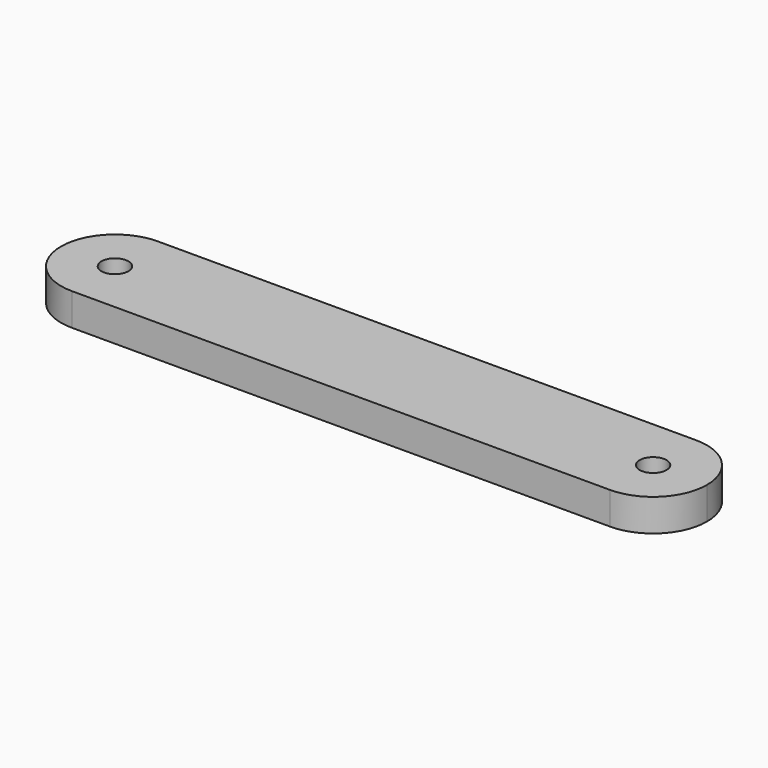
from build123d import *

# Parameters (mm, degrees)
F0_W     = 30.48
F0_H     = 5.08
F0_R     = 0.635
F1_DEPTH = 1.524
F2_R     = 2.53999


# Not quite as in the source:
# - a fillet or chamfer is up to 0.001 mm smaller than in the source, because OpenCascade refuses the exact size


with BuildPart() as f1:
    # F0 (on Top) → F1 (new body)
    with BuildSketch(Plane.XY):
        with Locations((15.24, 2.54)):
            Rectangle(F0_W, F0_H)
        with Locations((2.54, 2.54)):
            Circle(F0_R, mode=Mode.SUBTRACT)
        with Locations((27.94, 2.54)):
            Circle(F0_R, mode=Mode.SUBTRACT)
    extrude(amount=F1_DEPTH)

    # F2 (radius 2.54 in the source; OpenCascade refuses exactly that, so slightly less here)
    f2_edges = [f1.edges().sort_by_distance(p)[0] for p in [
        (0, 0, 0.762),
        (0, 5.08, 0.762),
        (30.48, 0, 0.762),
        (30.48, 5.08, 0.762),
    ]]
    fillet(f2_edges, radius=F2_R)


solid = f1.part
